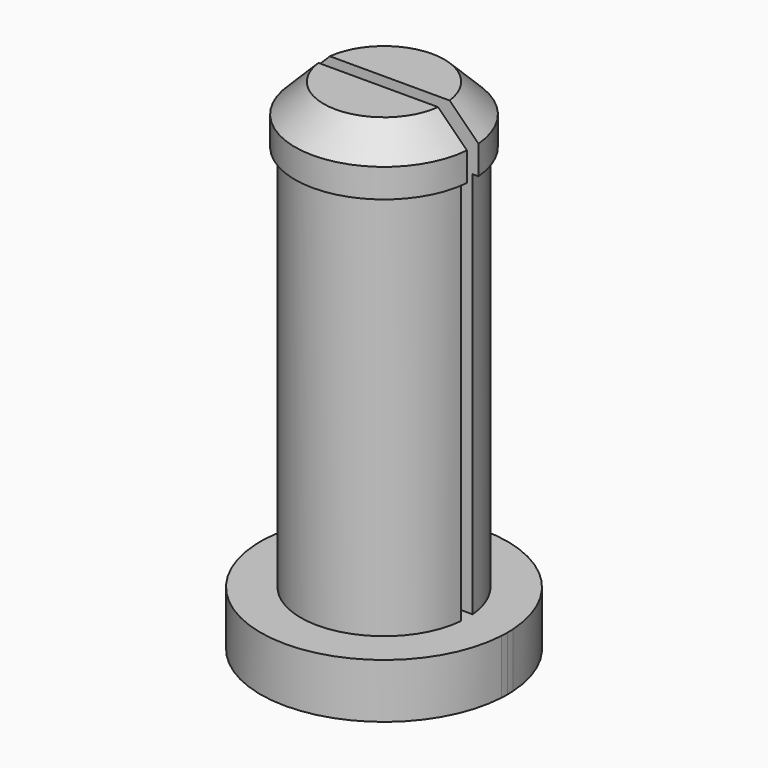
from build123d import *

# Parameters (mm, degrees)
F1_DEPTH = 1.9
F2_DEPTH = 13.5
F4_DEPTH = 2
F5_SIZE  = 1


with BuildPart() as f1:
    # F0 (on Top) → F1 (new body)
    with BuildSketch(Plane.XY):
        with BuildLine():
            Line((2.8892040426, 0.25), (4.2927264064, 0.25))
            ThreePointArc((4.2927264064, 0.25), (0, 4.3), (-4.2927264064, 0.25))
            Line((-4.2927264064, 0.25), (-2.8892040426, 0.25))
            ThreePointArc((-2.8892040426, 0.25), (0, 2.9), (2.8892040426, 0.25))
        make_face()
        with BuildLine():
            Line((0, 0.25), (2.8892040426, 0.25))
            ThreePointArc((2.8892040426, 0.25), (0, 2.9), (-2.8892040426, 0.25))
            Line((-2.8892040426, 0.25), (0, 0.25))
        make_face()
        with BuildLine():
            Line((-2.8892040426, 0.25), (-4.2927264064, 0.25))
            ThreePointArc((-4.2927264064, 0.25), (-4.3, 0), (-4.2927264064, -0.25))
            Line((-4.2927264064, -0.25), (-2.8892040426, -0.25))
            ThreePointArc((-2.8892040426, -0.25), (-2.9, 0), (-2.8892040426, 0.25))
        make_face()
        with BuildLine():
            ThreePointArc((4.2927264064, -0.25), (4.2981812169, -0.125052894), (4.3, 0))
            ThreePointArc((4.3, 0), (4.2981812169, 0.125052894), (4.2927264064, 0.25))
            Line((4.2927264064, 0.25), (2.8892040426, 0.25))
            ThreePointArc((2.8892040426, 0.25), (2.8972997535, 0.1251164984), (2.9, 0))
            ThreePointArc((2.9, 0), (2.8972997535, -0.1251164984), (2.8892040426, -0.25))
            Line((2.8892040426, -0.25), (4.2927264064, -0.25))
        make_face()
        with BuildLine():
            ThreePointArc((-4.2927264064, -0.25), (0, -4.3), (4.2927264064, -0.25))
            Line((4.2927264064, -0.25), (2.8892040426, -0.25))
            ThreePointArc((2.8892040426, -0.25), (0, -2.9), (-2.8892040426, -0.25))
            Line((-2.8892040426, -0.25), (-4.2927264064, -0.25))
        make_face()
        with BuildLine():
            ThreePointArc((-2.8892040426, -0.25), (0, -2.9), (2.8892040426, -0.25))
            Line((2.8892040426, -0.25), (0, -0.25))
            Line((0, -0.25), (-2.8892040426, -0.25))
        make_face()
        with BuildLine():
            ThreePointArc((2.9, 0), (2.8972997535, 0.1251164984), (2.8892040426, 0.25))
            Line((2.8892040426, 0.25), (0, 0.25))
            Line((0, 0.25), (-2.8892040426, 0.25))
            ThreePointArc((-2.8892040426, 0.25), (-2.9, 0), (-2.8892040426, -0.25))
            Line((-2.8892040426, -0.25), (0, -0.25))
            Line((0, -0.25), (2.8892040426, -0.25))
            ThreePointArc((2.8892040426, -0.25), (2.8972997535, -0.1251164984), (2.9, 0))
        make_face()
    extrude(amount=-F1_DEPTH)

    # F0 (on Top) → F2 (join)
    with BuildSketch(Plane.XY):
        with BuildLine():
            ThreePointArc((-2.8892040426, -0.25), (0, -2.9), (2.8892040426, -0.25))
            Line((2.8892040426, -0.25), (0, -0.25))
            Line((0, -0.25), (-2.8892040426, -0.25))
        make_face()
        with BuildLine():
            Line((0, 0.25), (2.8892040426, 0.25))
            ThreePointArc((2.8892040426, 0.25), (0, 2.9), (-2.8892040426, 0.25))
            Line((-2.8892040426, 0.25), (0, 0.25))
        make_face()
    extrude(amount=F2_DEPTH)

    # F3 (on face) → F4 (join)
    with BuildSketch(Plane.XY.offset(13.5)):
        with BuildLine():
            ThreePointArc((-3.0899029111, -0.25), (0, -3.1), (3.0899029111, -0.25))
            Line((3.0899029111, -0.25), (0, -0.25))
            Line((0, -0.25), (-3.0899029111, -0.25))
        make_face()
        with BuildLine():
            Line((0, 0.25), (2.8892040426, 0.25))
            ThreePointArc((2.8892040426, 0.25), (0, 2.9), (-2.8892040426, 0.25))
            Line((-2.8892040426, 0.25), (0, 0.25))
        make_face()
        with BuildLine():
            Line((2.8892040426, 0.25), (3.0899029111, 0.25))
            ThreePointArc((3.0899029111, 0.25), (0, 3.1), (-3.0899029111, 0.25))
            Line((-3.0899029111, 0.25), (-2.8892040426, 0.25))
            ThreePointArc((-2.8892040426, 0.25), (0, 2.9), (2.8892040426, 0.25))
        make_face()
    extrude(amount=F4_DEPTH)

    # F5
    f5_edges = [f1.edges().sort_by_distance(p)[0] for p in [
        (0, 3.1, 15.5),
        (0, -3.1, 15.5),
    ]]
    chamfer(f5_edges, length=F5_SIZE)


solid = f1.part
